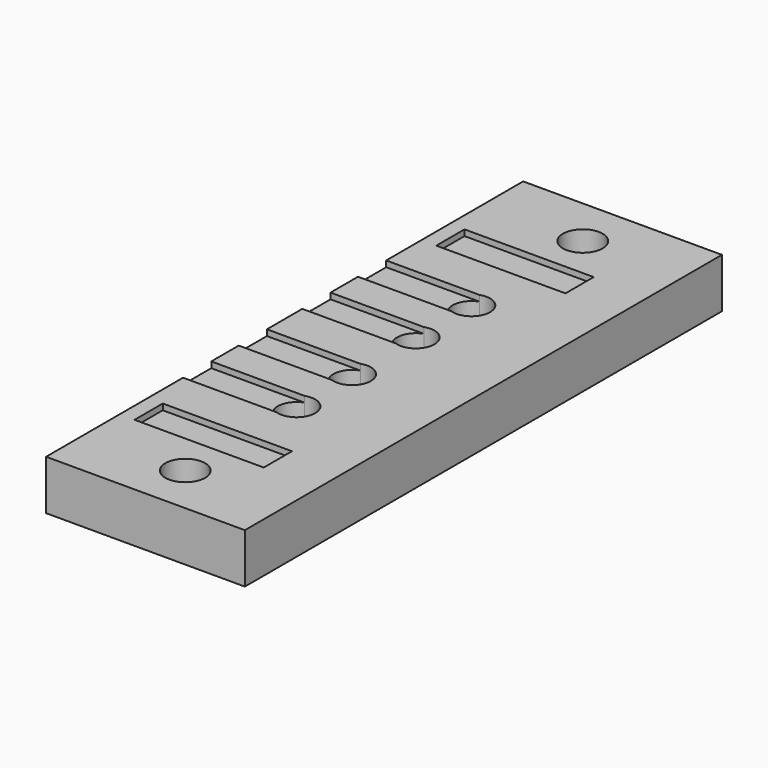
from build123d import *

# Parameters (mm, degrees)
F0_W     = 26
F0_H     = 7.1
F0_R     = 4
F1_DEPTH = 10
F2_DEPTH = 1.2
F3_DEPTH = 4.2


# Not quite as in the source:
# - a feature names something its author has since deleted; it is built from what else it names


with BuildPart() as f1:
    # F0 (on Top) → F1 (new body)
    with BuildSketch(Plane.XY):
        with BuildLine():
            Line((-20, -60), (20, -60))
            Line((20, -60), (20, 60))
            Line((20, 60), (-20, 60))
            Line((-20, 60), (-20, 25.55))
            Line((-20, 25.55), (-1.2083045974, 25.55))
            ThreePointArc((-1.2083045974, 25.55), (2.1830434902, 25.0490688939), (3.75, 22))
            ThreePointArc((3.75, 22), (2.1830434902, 18.9509311061), (-1.2083045974, 18.45))
            Line((-1.2083045974, 18.45), (-20, 18.45))
            Line((-20, 18.45), (-20, 11.55))
            Line((-20, 11.55), (-1.2083045974, 11.55))
            ThreePointArc((-1.2083045974, 11.55), (2.1830434902, 11.0490688939), (3.75, 8))
            ThreePointArc((3.75, 8), (2.1830434902, 4.9509311061), (-1.2083045974, 4.45))
            Line((-1.2083045974, 4.45), (-20, 4.45))
            Line((-20, 4.45), (-20, -4.45))
            Line((-20, -4.45), (-1.2083045974, -4.45))
            ThreePointArc((-1.2083045974, -4.45), (2.1830434902, -4.9509311061), (3.75, -8))
            ThreePointArc((3.75, -8), (2.1830434902, -11.0490688939), (-1.2083045974, -11.55))
            Line((-1.2083045974, -11.55), (-20, -11.55))
            Line((-20, -11.55), (-20, -18.45))
            Line((-20, -18.45), (-1.2083045974, -18.45))
            ThreePointArc((-1.2083045974, -18.45), (2.1830434902, -18.9509311061), (3.75, -22))
            ThreePointArc((3.75, -22), (2.1830434902, -25.0490688939), (-1.2083045974, -25.55))
            Line((-1.2083045974, -25.55), (-20, -25.55))
            Line((-20, -25.55), (-20, -60))
        make_face()
        with Locations((-4, -37.95)):
            Rectangle(F0_W, F0_H, mode=Mode.SUBTRACT)
        with Locations((0, -50)):
            Circle(F0_R, mode=Mode.SUBTRACT)
        with Locations((-4, 37.95)):
            Rectangle(F0_W, F0_H, mode=Mode.SUBTRACT)
        with Locations((0, 50)):
            Circle(F0_R, mode=Mode.SUBTRACT)
        with BuildLine():
            Line((-20, -18.45), (-20, -25.55))
            Line((-20, -25.55), (-1.2083045974, -25.55))
            ThreePointArc((-1.2083045974, -25.55), (-3.75, -22), (-1.2083045974, -18.45))
            Line((-1.2083045974, -18.45), (-20, -18.45))
        make_face()
        with BuildLine():
            Line((-1.2083045974, 25.55), (-20, 25.55))
            Line((-20, 25.55), (-20, 18.45))
            Line((-20, 18.45), (-1.2083045974, 18.45))
            ThreePointArc((-1.2083045974, 18.45), (-3.75, 22), (-1.2083045974, 25.55))
        make_face()
        with BuildLine():
            Line((-20, -4.45), (-20, -11.55))
            Line((-20, -11.55), (-1.2083045974, -11.55))
            ThreePointArc((-1.2083045974, -11.55), (-3.75, -8), (-1.2083045974, -4.45))
            Line((-1.2083045974, -4.45), (-20, -4.45))
        make_face()
        with BuildLine():
            Line((-1.2083045974, 11.55), (-20, 11.55))
            Line((-20, 11.55), (-20, 4.45))
            Line((-20, 4.45), (-1.2083045974, 4.45))
            ThreePointArc((-1.2083045974, 4.45), (-3.75, 8), (-1.2083045974, 11.55))
        make_face()
        with BuildLine():
            Line((0, 25.55), (-1.2083045974, 25.55))
            ThreePointArc((-1.2083045974, 25.55), (-3.75, 22), (-1.2083045974, 18.45))
            Line((-1.2083045974, 18.45), (0, 18.45))
            Line((0, 18.45), (0, 20.25))
            ThreePointArc((0, 20.25), (-1.75, 22), (0, 23.75))
            Line((0, 23.75), (0, 25.55))
        make_face()
        with BuildLine():
            ThreePointArc((3.75, 22), (2.1830434902, 25.0490688939), (-1.2083045974, 25.55))
            Line((-1.2083045974, 25.55), (0, 25.55))
            Line((0, 25.55), (0, 23.75))
            ThreePointArc((0, 23.75), (1.2374368671, 23.2374368671), (1.75, 22))
            ThreePointArc((1.75, 22), (1.2374368671, 20.7625631329), (0, 20.25))
            Line((0, 20.25), (0, 18.45))
            Line((0, 18.45), (-1.2083045974, 18.45))
            ThreePointArc((-1.2083045974, 18.45), (2.1830434902, 18.9509311061), (3.75, 22))
        make_face()
        with BuildLine():
            ThreePointArc((3.75, 8), (2.1830434902, 11.0490688939), (-1.2083045974, 11.55))
            Line((-1.2083045974, 11.55), (0, 11.55))
            Line((0, 11.55), (0, 9.75))
            ThreePointArc((0, 9.75), (1.2374368671, 9.2374368671), (1.75, 8))
            ThreePointArc((1.75, 8), (1.2374368671, 6.7625631329), (0, 6.25))
            Line((0, 6.25), (0, 4.45))
            Line((0, 4.45), (-1.2083045974, 4.45))
            ThreePointArc((-1.2083045974, 4.45), (2.1830434902, 4.9509311061), (3.75, 8))
        make_face()
        with BuildLine():
            Line((0, 11.55), (-1.2083045974, 11.55))
            ThreePointArc((-1.2083045974, 11.55), (-3.75, 8), (-1.2083045974, 4.45))
            Line((-1.2083045974, 4.45), (0, 4.45))
            Line((0, 4.45), (0, 6.25))
            ThreePointArc((0, 6.25), (-1.75, 8), (0, 9.75))
            Line((0, 9.75), (0, 11.55))
        make_face()
        with BuildLine():
            ThreePointArc((-1.2083045974, -4.45), (-3.75, -8), (-1.2083045974, -11.55))
            Line((-1.2083045974, -11.55), (0, -11.55))
            Line((0, -11.55), (0, -9.75))
            ThreePointArc((0, -9.75), (-1.75, -8), (0, -6.25))
            Line((0, -6.25), (0, -4.45))
            Line((0, -4.45), (-1.2083045974, -4.45))
        make_face()
        with BuildLine():
            Line((0, -11.55), (-1.2083045974, -11.55))
            ThreePointArc((-1.2083045974, -11.55), (2.1830434902, -11.0490688939), (3.75, -8))
            ThreePointArc((3.75, -8), (2.1830434902, -4.9509311061), (-1.2083045974, -4.45))
            Line((-1.2083045974, -4.45), (0, -4.45))
            Line((0, -4.45), (0, -6.25))
            ThreePointArc((0, -6.25), (1.2374368671, -6.7625631329), (1.75, -8))
            ThreePointArc((1.75, -8), (1.2374368671, -9.2374368671), (0, -9.75))
            Line((0, -9.75), (0, -11.55))
        make_face()
        with BuildLine():
            Line((0, -25.55), (-1.2083045974, -25.55))
            ThreePointArc((-1.2083045974, -25.55), (2.1830434902, -25.0490688939), (3.75, -22))
            ThreePointArc((3.75, -22), (2.1830434902, -18.9509311061), (-1.2083045974, -18.45))
            Line((-1.2083045974, -18.45), (0, -18.45))
            Line((0, -18.45), (0, -20.25))
            ThreePointArc((0, -20.25), (1.2374368671, -20.7625631329), (1.75, -22))
            ThreePointArc((1.75, -22), (1.2374368671, -23.2374368671), (0, -23.75))
            Line((0, -23.75), (0, -25.55))
        make_face()
        with BuildLine():
            ThreePointArc((-1.2083045974, -18.45), (-3.75, -22), (-1.2083045974, -25.55))
            Line((-1.2083045974, -25.55), (0, -25.55))
            Line((0, -25.55), (0, -23.75))
            ThreePointArc((0, -23.75), (-1.75, -22), (0, -20.25))
            Line((0, -20.25), (0, -18.45))
            Line((0, -18.45), (-1.2083045974, -18.45))
        make_face()
        with Locations((-4, 37.95)):
            Rectangle(F0_W, F0_H)
        with Locations((-4, -37.95)):
            Rectangle(F0_W, F0_H)
    extrude(amount=-F1_DEPTH)

    # F0 (on Top) → F2 (cut)
    with BuildSketch(Plane.XY):
        with BuildLine():
            Line((-1.2083045974, 25.55), (-20, 25.55))
            Line((-20, 25.55), (-20, 18.45))
            Line((-20, 18.45), (-1.2083045974, 18.45))
            ThreePointArc((-1.2083045974, 18.45), (-3.75, 22), (-1.2083045974, 25.55))
        make_face()
        with BuildLine():
            Line((-1.2083045974, 11.55), (-20, 11.55))
            Line((-20, 11.55), (-20, 4.45))
            Line((-20, 4.45), (-1.2083045974, 4.45))
            ThreePointArc((-1.2083045974, 4.45), (-3.75, 8), (-1.2083045974, 11.55))
        make_face()
        with BuildLine():
            Line((-20, -4.45), (-20, -11.55))
            Line((-20, -11.55), (-1.2083045974, -11.55))
            ThreePointArc((-1.2083045974, -11.55), (-3.75, -8), (-1.2083045974, -4.45))
            Line((-1.2083045974, -4.45), (-20, -4.45))
        make_face()
        with BuildLine():
            Line((-20, -18.45), (-20, -25.55))
            Line((-20, -25.55), (-1.2083045974, -25.55))
            ThreePointArc((-1.2083045974, -25.55), (-3.75, -22), (-1.2083045974, -18.45))
            Line((-1.2083045974, -18.45), (-20, -18.45))
        make_face()
        with Locations((-4, 37.95)):
            Rectangle(F0_W, F0_H)
        with Locations((-4, -37.95)):
            Rectangle(F0_W, F0_H)
    extrude(amount=-F2_DEPTH, mode=Mode.SUBTRACT)

    # F0 (on Top) → F3 (cut)
    with BuildSketch(Plane.XY):
        with BuildLine():
            Line((0, 25.55), (-1.2083045974, 25.55))
            ThreePointArc((-1.2083045974, 25.55), (-3.75, 22), (-1.2083045974, 18.45))
            Line((-1.2083045974, 18.45), (0, 18.45))
            Line((0, 18.45), (0, 20.25))
            ThreePointArc((0, 20.25), (-1.75, 22), (0, 23.75))
            Line((0, 23.75), (0, 25.55))
        make_face()
        with BuildLine():
            ThreePointArc((3.75, 22), (2.1830434902, 25.0490688939), (-1.2083045974, 25.55))
            Line((-1.2083045974, 25.55), (0, 25.55))
            Line((0, 25.55), (0, 23.75))
            ThreePointArc((0, 23.75), (1.2374368671, 23.2374368671), (1.75, 22))
            ThreePointArc((1.75, 22), (1.2374368671, 20.7625631329), (0, 20.25))
            Line((0, 20.25), (0, 18.45))
            Line((0, 18.45), (-1.2083045974, 18.45))
            ThreePointArc((-1.2083045974, 18.45), (2.1830434902, 18.9509311061), (3.75, 22))
        make_face()
        with BuildLine():
            Line((0, 11.55), (-1.2083045974, 11.55))
            ThreePointArc((-1.2083045974, 11.55), (-3.75, 8), (-1.2083045974, 4.45))
            Line((-1.2083045974, 4.45), (0, 4.45))
            Line((0, 4.45), (0, 6.25))
            ThreePointArc((0, 6.25), (-1.75, 8), (0, 9.75))
            Line((0, 9.75), (0, 11.55))
        make_face()
        with BuildLine():
            ThreePointArc((3.75, 8), (2.1830434902, 11.0490688939), (-1.2083045974, 11.55))
            Line((-1.2083045974, 11.55), (0, 11.55))
            Line((0, 11.55), (0, 9.75))
            ThreePointArc((0, 9.75), (1.2374368671, 9.2374368671), (1.75, 8))
            ThreePointArc((1.75, 8), (1.2374368671, 6.7625631329), (0, 6.25))
            Line((0, 6.25), (0, 4.45))
            Line((0, 4.45), (-1.2083045974, 4.45))
            ThreePointArc((-1.2083045974, 4.45), (2.1830434902, 4.9509311061), (3.75, 8))
        make_face()
        with BuildLine():
            ThreePointArc((-1.2083045974, -4.45), (-3.75, -8), (-1.2083045974, -11.55))
            Line((-1.2083045974, -11.55), (0, -11.55))
            Line((0, -11.55), (0, -9.75))
            ThreePointArc((0, -9.75), (-1.75, -8), (0, -6.25))
            Line((0, -6.25), (0, -4.45))
            Line((0, -4.45), (-1.2083045974, -4.45))
        make_face()
        with BuildLine():
            Line((0, -11.55), (-1.2083045974, -11.55))
            ThreePointArc((-1.2083045974, -11.55), (2.1830434902, -11.0490688939), (3.75, -8))
            ThreePointArc((3.75, -8), (2.1830434902, -4.9509311061), (-1.2083045974, -4.45))
            Line((-1.2083045974, -4.45), (0, -4.45))
            Line((0, -4.45), (0, -6.25))
            ThreePointArc((0, -6.25), (1.2374368671, -6.7625631329), (1.75, -8))
            ThreePointArc((1.75, -8), (1.2374368671, -9.2374368671), (0, -9.75))
            Line((0, -9.75), (0, -11.55))
        make_face()
        with BuildLine():
            Line((0, -25.55), (-1.2083045974, -25.55))
            ThreePointArc((-1.2083045974, -25.55), (2.1830434902, -25.0490688939), (3.75, -22))
            ThreePointArc((3.75, -22), (2.1830434902, -18.9509311061), (-1.2083045974, -18.45))
            Line((-1.2083045974, -18.45), (0, -18.45))
            Line((0, -18.45), (0, -20.25))
            ThreePointArc((0, -20.25), (1.2374368671, -20.7625631329), (1.75, -22))
            ThreePointArc((1.75, -22), (1.2374368671, -23.2374368671), (0, -23.75))
            Line((0, -23.75), (0, -25.55))
        make_face()
        with BuildLine():
            ThreePointArc((-1.2083045974, -18.45), (-3.75, -22), (-1.2083045974, -25.55))
            Line((-1.2083045974, -25.55), (0, -25.55))
            Line((0, -25.55), (0, -23.75))
            ThreePointArc((0, -23.75), (-1.75, -22), (0, -20.25))
            Line((0, -20.25), (0, -18.45))
            Line((0, -18.45), (-1.2083045974, -18.45))
        make_face()
    extrude(amount=-F3_DEPTH, mode=Mode.SUBTRACT)


solid = f1.part
